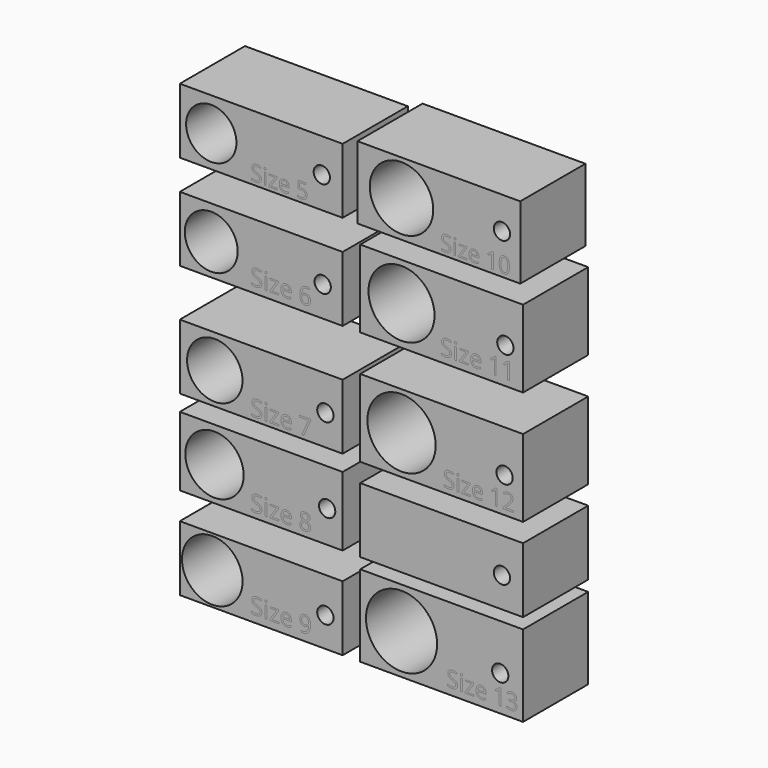
from build123d import *

# Parameters (mm, degrees)
F0_W           = 50.8
F0_H           = 20.32
F0_R           = 7.85
F0_R_2         = 2.54
F2_DEPTH       = 25.4
F0_R_3         = 8.25
F0_R_4         = 8.65
F0_H_2         = 21.59
F0_R_5         = 9.1
F0_R_6         = 9.45
F0_H_3         = 22.606
F0_R_7         = 9.9
F0_H_4         = 24.13
F0_R_8         = 10.3
F0_R_9         = 10.65
F0_H_5         = 25.4
F0_R_10        = 11.1
F1_TEXT_SIZE   = 6.7911694401
F1_TEXT_SIZE_2 = 7.1730174984
F1_TEXT_SIZE_3 = 7.1784614372
F1_TEXT_SIZE_4 = 7.1809768123
F1_TEXT_SIZE_5 = 7.1860128547
F1_TEXT_SIZE_6 = 6.9401420963
F1_TEXT_SIZE_7 = 6.940557311
F3_DEPTH       = 25.4


# Not quite as in the source:
# - Text() gives the source's letters only with a copy of the font that has no kerning and outlines rounded to 1/6400 em; it was checked with that copy


with BuildPart() as f2:
    # F0 (on Front) → F2 (new body)
    with BuildSketch(Plane.XZ):
        with Locations((-43.7635087132, 60.068105284)):
            Rectangle(F0_W, F0_H)
        with Locations((-59.3533739448, 59.7665049136)):
            Circle(F0_R, mode=Mode.SUBTRACT)
        with Locations((-24.8668286949, 59.6221126616)):
            Circle(F0_R_2, mode=Mode.SUBTRACT)
    extrude(amount=F2_DEPTH)


with BuildPart() as f2b:
    # F0 (on Front) → F2, piece 2 (new body)
    with BuildSketch(Plane.XZ):
        with Locations((-43.7635087132, 30.37551691)):
            Rectangle(F0_W, F0_H)
        with Locations((-59.3533739448, 30.0209634006)):
            Circle(F0_R_3, mode=Mode.SUBTRACT)
        with Locations((-24.5889890939, 29.6152122319)):
            Circle(F0_R_2, mode=Mode.SUBTRACT)
    extrude(amount=F2_DEPTH)


with BuildPart() as f2c:
    # F0 (on Front) → F2, piece 3 (new body)
    with BuildSketch(Plane.XZ):
        with Locations((-43.7635087132, -4.7127707565)):
            Rectangle(F0_W, F0_H)
        with Locations((-58.2516901195, -4.9575907178)):
            Circle(F0_R_4, mode=Mode.SUBTRACT)
        with Locations((-23.7554647028, -5.3928401321)):
            Circle(F0_R_2, mode=Mode.SUBTRACT)
    extrude(amount=F2_DEPTH)


with BuildPart() as f2d:
    # F0 (on Front) → F2, piece 4 (new body)
    with BuildSketch(Plane.XZ):
        with Locations((-43.7635087132, -30.6802773941)):
            Rectangle(F0_W, F0_H_2)
        with Locations((-58.3483055234, -30.8794360608)):
            Circle(F0_R_5, mode=Mode.SUBTRACT)
        with Locations((-23.1997799128, -31.5099582076)):
            Circle(F0_R_2, mode=Mode.SUBTRACT)
    extrude(amount=F2_DEPTH)


with BuildPart() as f2e:
    # F0 (on Front) → F2, piece 5 (new body)
    with BuildSketch(Plane.XZ):
        with Locations((-43.7635087132, -60.0725329185)):
            Rectangle(F0_W, F0_H)
        with Locations((-59.0413585305, -60.1276531816)):
            Circle(F0_R_6, mode=Mode.SUBTRACT)
        with Locations((-23.7554647028, -60.96117571)):
            Circle(F0_R_2, mode=Mode.SUBTRACT)
    extrude(amount=F2_DEPTH)


with BuildPart() as f2f:
    # F0 (on Front) → F2, piece 6 (new body)
    with BuildSketch(Plane.XZ):
        with Locations((11.6427292392, 61.1543281345)):
            Rectangle(F0_W, F0_H_3)
        with Locations((0, 61.289165169)):
            Circle(F0_R_7, mode=Mode.SUBTRACT)
        with Locations((31.3183031976, 62.3702071607)):
            Circle(F0_R_2, mode=Mode.SUBTRACT)
    extrude(amount=F2_DEPTH)


with BuildPart() as f2g:
    # F0 (on Front) → F2, piece 7 (new body)
    with BuildSketch(Plane.XZ):
        with Locations((12.5143829077, 32.28051691)):
            Rectangle(F0_W, F0_H_4)
        with Locations((0, 32.393630594)):
            Circle(F0_R_8, mode=Mode.SUBTRACT)
        with Locations((32.3896660352, 31.4168495306)):
            Circle(F0_R_2, mode=Mode.SUBTRACT)
    extrude(amount=F2_DEPTH)


with BuildPart() as f2h:
    # F0 (on Front) → F2, piece 8 (new body)
    with BuildSketch(Plane.XZ):
        with Locations((12.5143829077, -3.2452790937)):
            Rectangle(F0_W, F0_H_4)
        with Locations((0, -3.1701067928)):
            Circle(F0_R_9, mode=Mode.SUBTRACT)
        with Locations((32.1527048945, -4.3166284449)):
            Circle(F0_R_2, mode=Mode.SUBTRACT)
    extrude(amount=F2_DEPTH)


with BuildPart() as f2i:
    # F0 (on Front) → F2, piece 9 (new body)
    with BuildSketch(Plane.XZ):
        with Locations((12.5143829077, -31.3152773941)):
            Rectangle(F0_W, F0_H)
        with Locations((31.3197635114, -32.1038626134)):
            Circle(F0_R_2, mode=Mode.SUBTRACT)
    extrude(amount=F2_DEPTH)


with BuildPart() as f2j:
    # F0 (on Front) → F2, piece 10 (new body)
    with BuildSketch(Plane.XZ):
        with Locations((12.5143829077, -57.5325329185)):
            Rectangle(F0_W, F0_H_5)
        with Locations((0, -57.6270744205)):
            Circle(F0_R_10, mode=Mode.SUBTRACT)
        with Locations((30.7968147099, -59.1357909143)):
            Circle(F0_R_2, mode=Mode.SUBTRACT)
    extrude(amount=F2_DEPTH)


with BuildPart() as f3:
    # F1 (on Front) → F3 (new body)
    with BuildSketch(Plane.XZ):
        with Locations((-47.1260133347, 50.9258540736)):
            Text('Size 5', F1_TEXT_SIZE, font='Open Sans', text_align=(TextAlign.LEFT, TextAlign.BOTTOM))
        with Locations((-47.1260133347, 22.1706965927)):
            Text('Size 6', F1_TEXT_SIZE_2, font='Open Sans', text_align=(TextAlign.LEFT, TextAlign.BOTTOM))
        with Locations((-47.1260133347, -13.783871283)):
            Text('Size 7', F1_TEXT_SIZE_3, font='Open Sans', text_align=(TextAlign.LEFT, TextAlign.BOTTOM))
        with Locations((-47.1260133347, -39.9015939798)):
            Text('Size 8', F1_TEXT_SIZE_4, font='Open Sans', text_align=(TextAlign.LEFT, TextAlign.BOTTOM))
        with Locations((-47.1260133347, -68.0574266352)):
            Text('Size 9', F1_TEXT_SIZE_5, font='Open Sans', text_align=(TextAlign.LEFT, TextAlign.BOTTOM))
        with Locations((12.0527010831, 50.9258540736)):
            Text('Size 10', F1_TEXT_SIZE, font='Open Sans', text_align=(TextAlign.LEFT, TextAlign.BOTTOM))
        with Locations((12.0527010831, 22.1706965927)):
            Text('Size 11', F1_TEXT_SIZE_2, font='Open Sans', text_align=(TextAlign.LEFT, TextAlign.BOTTOM))
        with Locations((12.9181463271, -13.728749007)):
            Text('Size 12', F1_TEXT_SIZE_6, font='Open Sans', text_align=(TextAlign.LEFT, TextAlign.BOTTOM))
        with Locations((14.0295885503, -68.2000741363)):
            Text('Size 13', F1_TEXT_SIZE_7, font='Open Sans', text_align=(TextAlign.LEFT, TextAlign.BOTTOM))
    extrude(amount=F3_DEPTH)


solid = Compound([f2.part, f2b.part, f2c.part, f2d.part, f2e.part, f2f.part, f2g.part, f2h.part, f2i.part, f2j.part, f3.part])
